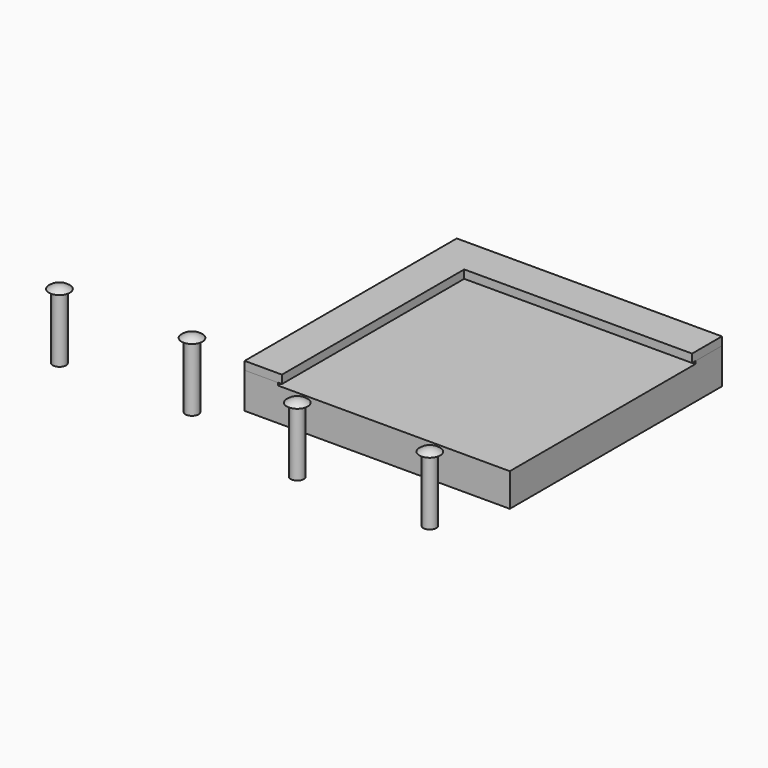
from build123d import *

# Parameters (mm, degrees)
F0_W      = 101.6
F0_H      = 101.6
F1_DEPTH  = 12.7
F3_DEPTH  = 1
F5_DEPTH  = 3.175
F7_W      = 2.25
F7_H      = 25
F10_COUNT = 2
F10_ANGLE = 90


# Not quite as in the source:
# - a length typed as a fraction of an inch, garbled in the dataset ("3 / 203.2 mm" for 3/8 in), is restored


with BuildPart() as f1:
    # F0 (on Top) → F1 (new body)
    with BuildSketch(Plane.XY):
        Rectangle(F0_W, F0_H)
    extrude(amount=F1_DEPTH)

    # F2 (on face) → F3 (join)
    with BuildSketch(Plane.XY.offset(12.7)):
        with BuildLine():
            Line((-50.8, -50.8), (-38.1, -50.8))
            Line((-38.1, -50.8), (-38.1, 36.5125))
            ThreePointArc((-38.1, 36.5125), (-39.2225320151, 39.2225320151), (-36.5125, 38.1))
            Line((-36.5125, 38.1), (50.8, 38.1))
            Line((50.8, 38.1), (50.8, 50.8))
            Line((50.8, 50.8), (-50.8, 50.8))
            Line((-50.8, 50.8), (-50.8, -50.8))
        make_face()
    extrude(amount=F3_DEPTH)


with BuildPart() as f5:
    # F4 (on face) → F5 (new body)
    with BuildSketch(Plane.XY.offset(13.7)):
        with BuildLine():
            Line((50.8, 38.1), (50.8, 50.8))
            Line((50.8, 50.8), (-50.8, 50.8))
            Line((-50.8, 50.8), (-50.8, -50.8))
            Line((-50.8, -50.8), (-38.1, -50.8))
            Line((-38.1, -50.8), (-38.1, 36.5125))
            ThreePointArc((-38.1, 36.5125), (-39.2225320151, 39.2225320151), (-36.5125, 38.1))
            Line((-36.5125, 38.1), (-34.925, 38.1))
            Line((-34.925, 38.1), (50.8, 38.1))
        make_face()
        with BuildLine():
            Line((50.8, 36.5125), (50.8, 38.1))
            Line((50.8, 38.1), (-34.925, 38.1))
            Line((-34.925, 38.1), (-36.5125, 38.1))
            ThreePointArc((-36.5125, 38.1), (-39.2225320151, 39.2225320151), (-38.1, 36.5125))
            Line((-38.1, 36.5125), (-38.1, -50.8))
            Line((-38.1, -50.8), (-36.5125, -50.8))
            Line((-36.5125, -50.8), (-36.5125, 36.5125))
            Line((-36.5125, 36.5125), (50.8, 36.5125))
        make_face()
    extrude(amount=F5_DEPTH)


with BuildPart() as f8:
    # F7 (on plane+point) → F8 (revolve)
    with BuildSketch(Plane.XZ.offset(-25.4)):
        with BuildLine():
            Line((-48.255014509, 13.7), (-46.755014509, 13.7))
            Line((-46.755014509, 13.7), (-46.755014509, -11.3))
            Line((-46.755014509, -11.3), (-46.505014509, -11.3))
            Line((-46.505014509, -11.3), (-46.505014509, 13.7))
            Line((-46.505014509, 13.7), (-44.255014509, 13.7))
            Line((-44.255014509, 13.7), (-44.255014509, 15.1545459404))
            ThreePointArc((-44.255014509, 15.1545459404), (-46.3831418485, 14.7796230362), (-48.255014509, 13.7))
        make_face()
        with Locations((-45.380014509, 1.2)):
            Rectangle(F7_W, F7_H)
    revolve(axis=Axis((-44.255014509, 25.4, 1.2), (0, 0, -1)))


with BuildPart() as f9_1:
    # F9: instance of F8
    add(f8.part.mirror(Plane.XZ))


with BuildPart() as f10_1:
    # F10: instance of F8
    add(f8.part.rotate(Axis((-50.8, -50.8, 6.35), (0, 0, -1)), 1 * F10_ANGLE / (F10_COUNT - 1)))


with BuildPart() as f10_2:
    # F10: instance of F8
    add(f8.part.rotate(Axis((-50.8, -50.8, 6.35), (0, 0, -1)), -1 * F10_ANGLE / (F10_COUNT - 1)))


with BuildPart() as f10_3:
    # F10: instance of F9_1
    add(f9_1.part.rotate(Axis((-50.8, -50.8, 6.35), (0, 0, -1)), 1 * F10_ANGLE / (F10_COUNT - 1)))


with BuildPart() as f10_4:
    # F10: instance of F9_1
    add(f9_1.part.rotate(Axis((-50.8, -50.8, 6.35), (0, 0, -1)), -1 * F10_ANGLE / (F10_COUNT - 1)))


solid = Compound([f1.part, f5.part, f8.part, f9_1.part, f10_1.part, f10_2.part, f10_3.part, f10_4.part])
